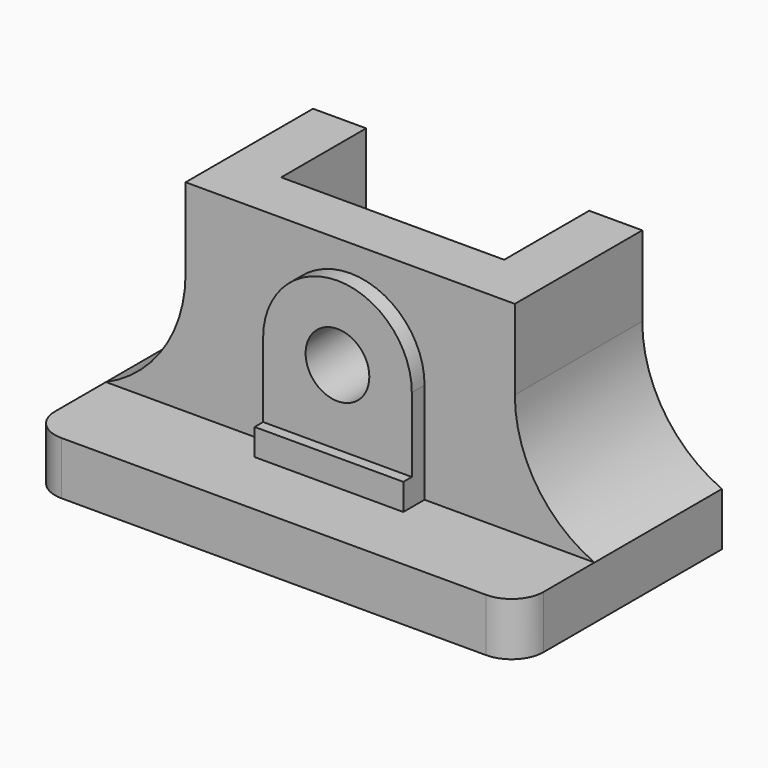
from build123d import *

# Parameters (mm, degrees)
F1_DEPTH = 48
F0_W     = 92
F0_H     = 18
F2_DEPTH = 10
F4_DEPTH = 63
F6_DEPTH = 5
F7_DEPTH = 3
F8_R     = 6
F9_DEPTH = 55.6
F10_R    = 6


with BuildPart() as f1:
    # F0 (on Top) → F1 (new body)
    with BuildSketch(Plane.XY):
        Polygon((-31, 29.8156050886), (-46, 29.8156050886), (-46, -0.1843949114), (46, -0.1843949114), (46, 29.8156050886), (31, 29.8156050886), (21, 29.8156050886), (21, 9.8156050886), (-21, 9.8156050886), (-21, 29.8156050886), align=None)
    extrude(amount=F1_DEPTH)

    # F0 (on Top) → F2 (join)
    with BuildSketch(Plane.XY):
        with Locations((0, -9.1843949114)):
            Rectangle(F0_W, F0_H)
    extrude(amount=F2_DEPTH)

    # F3 (on face) → F4 (cut)
    with BuildSketch(Plane.XZ.offset(0.1843949114)):
        with BuildLine():
            Line((-31, 32.9128784748), (-31, 48))
            Line((-31, 48), (-36.0656386086, 48))
            ThreePointArc((-36.0656386086, 48), (-32.3002211531, 40.8702953048), (-31, 32.9128784748))
        make_face()
        with BuildLine():
            ThreePointArc((-46, 10), (-35.0834993366, 19.2198145372), (-31, 32.9128784748))
            ThreePointArc((-31, 32.9128784748), (-32.3002211531, 40.8702953048), (-36.0656386086, 48))
            Line((-36.0656386086, 48), (-46, 48))
            Line((-46, 48), (-46, 10))
        make_face()
        with BuildLine():
            Line((36.0656386086, 48), (31, 48))
            Line((31, 48), (31, 32.9128784748))
            ThreePointArc((31, 32.9128784748), (32.3002211531, 40.8702953048), (36.0656386086, 48))
        make_face()
        with BuildLine():
            ThreePointArc((36.0656386086, 48), (32.3002211531, 40.8702953048), (31, 32.9128784748))
            ThreePointArc((31, 32.9128784748), (35.0834993366, 19.2198145372), (46, 10))
            Line((46, 10), (46, 48))
            Line((46, 48), (36.0656386086, 48))
        make_face()
        with BuildLine():
            ThreePointArc((81, 32.9128784748), (63.9574168301, 56.6126573217), (36.0656386086, 48))
            Line((36.0656386086, 48), (46, 48))
            Line((46, 48), (46, 10))
            ThreePointArc((46, 10), (69.6930639376, 11.9963778114), (81, 32.9128784748))
        make_face()
    extrude(amount=-F4_DEPTH, mode=Mode.SUBTRACT)

    # F5 (on face) → F6 (join)
    with BuildSketch(Plane.XZ.offset(0.1843949114)):
        Polygon((14, 15), (0, 15), (-14, 15), (-14, 10), (14, 10), align=None)
    extrude(amount=F6_DEPTH)

    # F5 (on face) → F7 (join)
    with BuildSketch(Plane.XZ.offset(0.1843949114)):
        with BuildLine():
            Line((0, 29), (14, 29))
            ThreePointArc((14, 29), (0, 43), (-14, 29))
            Line((-14, 29), (0, 29))
        make_face()
        with BuildLine():
            ThreePointArc((0, 15), (9.8994949366, 19.1005050634), (14, 29))
            Line((14, 29), (0, 29))
            Line((0, 29), (-14, 29))
            ThreePointArc((-14, 29), (-9.8994949366, 19.1005050634), (0, 15))
        make_face()
        with BuildLine():
            Line((14, 15), (14, 29))
            ThreePointArc((14, 29), (9.8994949366, 19.1005050634), (0, 15))
            Line((0, 15), (14, 15))
        make_face()
        with BuildLine():
            ThreePointArc((0, 15), (-9.8994949366, 19.1005050634), (-14, 29))
            Line((-14, 29), (-14, 15))
            Line((-14, 15), (0, 15))
        make_face()
    extrude(amount=F7_DEPTH)

    # F8 (on face) → F9 (cut)
    with BuildSketch(Plane.XZ.offset(3.1843949114)):
        with Locations((0, 29)):
            Circle(F8_R)
    extrude(amount=-F9_DEPTH, mode=Mode.SUBTRACT)

    # F10
    f10_edges = [f1.edges().sort_by_distance(p)[0] for p in [
        (-46, -18.184395, 5),
        (46, -18.184395, 5),
    ]]
    fillet(f10_edges, radius=F10_R)


solid = f1.part
